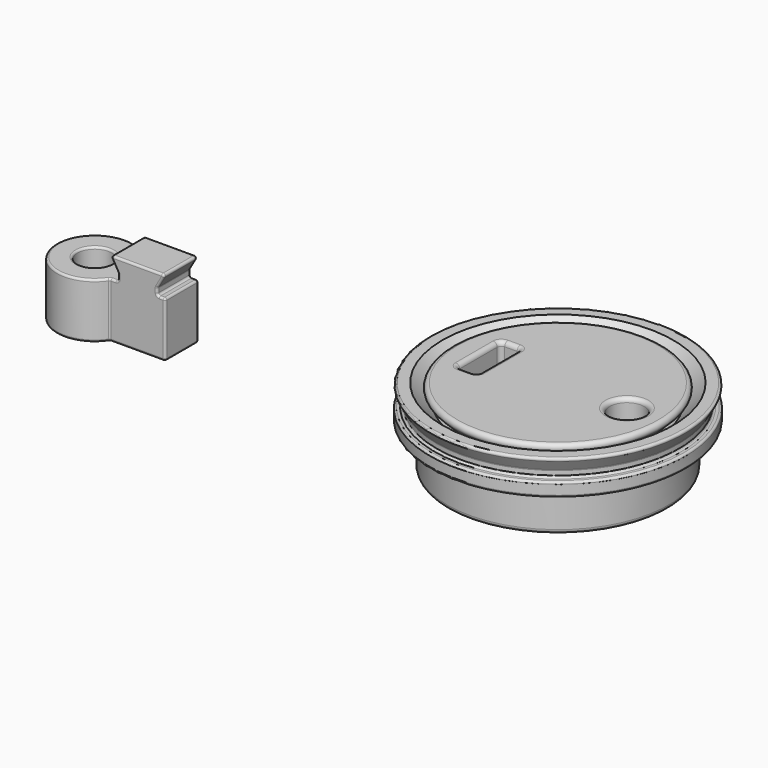
from build123d import *

# Parameters (mm, degrees)
F4_R      = 2.5
F5_DEPTH  = 11.001
F4_W      = 3
F4_H      = 8
F6_DEPTH  = 11.001
F7_R      = 0.5
F8_R      = 0.6
F9_R      = 0.3
F10_R     = 2.5
F11_DEPTH = 8
F12_W     = 8
F12_H     = 6
F13_DEPTH = 3
F15_DEPTH = 25.7509134082
F16_R     = 0.3


# Not quite as in the source:
# - a feature names something its author has since deleted; it is built from what else it names


with BuildPart() as f3:
    # F2 (on Front) → F3 (revolve)
    with BuildSketch(Plane.XZ):
        Polygon((-16, 0), (0, 0), (0, 11), (-16, 11), (-13.5, 8.5), (-16, 6), align=None)
    revolve(axis=Axis((0, 0, 5.5), (0, 0, 1)))

    # F4 (on face) → F5 (cut, through all)
    with BuildSketch(Plane.XY.offset(11)):
        with Locations((10, 0)):
            Circle(F4_R)
    extrude(amount=-F5_DEPTH, mode=Mode.SUBTRACT)

    # F4 (on face) → F6 (cut, through all)
    with BuildSketch(Plane.XY.offset(11)):
        with Locations((10, 0)):
            Circle(F4_R)
        with Locations((-10, 0)):
            Rectangle(F4_W, F4_H)
    extrude(amount=-F6_DEPTH, mode=Mode.SUBTRACT)

    # F7
    f7_edges = [f3.edges().sort_by_distance(p)[0] for p in [
        (7.5, 0, 0),
    ]]
    fillet(f7_edges, radius=F7_R)

    # F8
    f8_edges = [f3.edges().sort_by_distance(p)[0] for p in [
        (16, 0, 11),
        (-11.5, 0, 11),
        (-10, 4, 11),
        (-8.5, 0, 11),
        (-10, -4, 11),
        (7.5, 0, 11),
        (7, 0, 0),
        (16, 0, 0),
        (-10, -4, 0),
        (-8.5, 0, 0),
        (-10, 4, 0),
        (-11.5, 0, 0),
        (-11.5, 4, 5.5),
        (-8.5, 4, 5.5),
        (-8.5, -4, 5.5),
        (-11.5, -4, 5.5),
    ]]
    fillet(f8_edges, radius=F8_R)


with BuildPart() as f3b:
    # F2 (on Front) → F3, piece 2 (revolve)
    with BuildSketch(Plane.XZ):
        Polygon((-16.7071067812, 6), (-14.2071067812, 8.5), (-16.7071067812, 11), (-18.7071067812, 11), (-17.5524062428, 9), (-17.5524062428, 8), (-18.5524062428, 8), (-18.5524062428, 6), align=None)
    revolve(axis=Axis((0, 0, 5.5), (0, 0, 1)))

    # F9
    f9_edges = [f3b.edges().sort_by_distance(p)[0] for p in [
        (17.552406, 0, 9),
        (17.552406, 0, 8),
        (-17.552406, 0, 8.5),
        (18.552406, 0, 8),
        (18.552406, 0, 6),
        (-18.552406, 0, 7),
        (18.707107, 0, 11),
        (-18.129757, 0, 10),
    ]]
    fillet(f9_edges, radius=F9_R)


with BuildPart() as f11:
    # F10 (on Top) → F11 (new body)
    with BuildSketch(Plane.XY):
        with BuildLine():
            ThreePointArc((-59.0929749971, -7.1975071654), (-58.4299990212, -5.7621561264), (-58.2027472258, -4.1975071654))
            ThreePointArc((-58.2027472258, -4.1975071654), (-58.4299990212, -2.6328582044), (-59.0929749971, -1.1975071654))
            ThreePointArc((-59.0929749971, -1.1975071654), (-69.2027472258, -4.1975071654), (-59.0929749971, -7.1975071654))
        make_face()
        with Locations((-63.7027472258, -4.1975071654)):
            Circle(F10_R, mode=Mode.SUBTRACT)
        with BuildLine():
            ThreePointArc((-59.0929749971, -1.1975071654), (-58.4299990212, -2.6328582044), (-58.2027472258, -4.1975071654))
            ThreePointArc((-58.2027472258, -4.1975071654), (-58.4299990212, -5.7621561264), (-59.0929749971, -7.1975071654))
            Line((-59.0929749971, -7.1975071654), (-51.0929749971, -7.1975071654))
            Line((-51.0929749971, -7.1975071654), (-51.0929749971, -1.1975071654))
            Line((-51.0929749971, -1.1975071654), (-59.0929749971, -1.1975071654))
        make_face()
    extrude(amount=F11_DEPTH)

    # F12 (on face) → F13 (join)
    with BuildSketch(Plane.XY.offset(8)):
        with Locations((-55.0929749971, -4.1975071654)):
            Rectangle(F12_W, F12_H)
    extrude(amount=F13_DEPTH)

    # F14 (on face) → F15 (cut, through all)
    with BuildSketch(Plane.XZ.offset(7.1975071654)):
        Polygon((-59.0929749971, 11), (-59.0929749971, 8), (-57.9382744587, 8), (-57.9382744587, 9), align=None)
        Polygon((-52.2476755355, 9), (-52.2476755355, 8), (-51.0929749971, 8), (-51.0929749971, 11), align=None)
    extrude(amount=-F15_DEPTH, mode=Mode.SUBTRACT)

    # F16
    f16_edges = [f11.edges().sort_by_distance(p)[0] for p in [
        (-55.092975, -7.197507, 11),
        (-51.092975, -4.197507, 11),
        (-55.092975, -1.197507, 11),
        (-59.092975, -4.197507, 11),
        (-69.202747, -4.197507, 8),
        (-58.515625, -7.197507, 8),
        (-57.938274, -4.197507, 8),
        (-58.515625, -1.197507, 8),
        (-66.202747, -4.197507, 8),
        (-57.938274, -7.197507, 8.5),
        (-57.938274, -4.197507, 9),
        (-57.938274, -1.197507, 8.5),
        (-52.247676, -7.197507, 8.5),
        (-52.247676, -4.197507, 8),
        (-52.247676, -1.197507, 8.5),
        (-52.247676, -4.197507, 9),
        (-55.092975, -7.197507, 0),
        (-51.092975, -7.197507, 4),
        (-51.670325, -7.197507, 8),
        (-51.670325, -7.197507, 10),
        (-58.515625, -7.197507, 10),
        (-59.092975, -7.197507, 4),
        (-51.092975, -4.197507, 0),
        (-51.092975, -1.197507, 4),
        (-51.092975, -4.197507, 8),
        (-66.202747, -4.197507, 0),
        (-51.670325, -1.197507, 10),
        (-51.670325, -1.197507, 8),
        (-55.092975, -1.197507, 0),
        (-59.092975, -1.197507, 4),
        (-58.515625, -1.197507, 10),
        (-69.202747, -4.197507, 0),
    ]]
    fillet(f16_edges, radius=F16_R)


solid = Compound([f3.part, f3b.part, f11.part])
